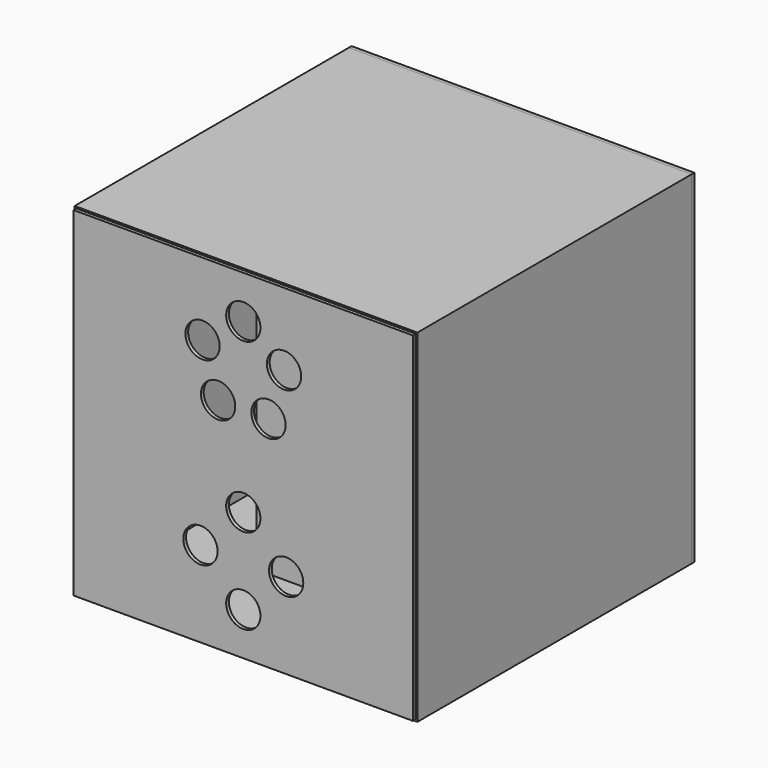
from build123d import *

# Parameters (mm, degrees)
F0_R      = 5.5
F1_DEPTH  = 19
F0_W      = 24.5
F0_H      = 25
F2_DEPTH  = 10
F3_DEPTH  = 60
F0_W_2    = 25
F0_H_2    = 0.5
F4_DEPTH  = 25
F5_D      = 10
F5_2_D    = 10
F5_3_D    = 10
F5_4_D    = 10
F5_5_D    = 10
F6_W      = 100
F6_H      = 100
F6_W_2    = 99
F6_H_2    = 99
F7_DEPTH  = 100
F8_W      = 99
F8_H      = 99
F8_R      = 5
F9_DEPTH  = 1
F10_W     = 100
F10_H     = 100
F11_DEPTH = 1
F13_R     = 5
F13_W     = 49.9103330076
F13_H     = 49.2593720555
F13_H_2   = 0.8928030729
F14_DEPTH = 5


# Not quite as in the source:
# - a pattern or mirror of a feature is missing from the dataset's text; its kind, count and spacing are read off the source's solid
# - a feature names something its author has since deleted; it is built from what else it names


with BuildPart() as f1:
    # F0 (on Front) → F1 (new body)
    with BuildSketch(Plane.XZ):
        with BuildLine():
            Line((-15.8034909498, 24.5), (-25, 24.5))
            Line((-25, 24.5), (-25, 0.5))
            Line((-25, 0.5), (0, 0.5))
            Line((0, 0.5), (0, 24.5))
            Line((0, 24.5), (-7.9729219576, 24.5))
            ThreePointArc((-7.9729219576, 24.5), (-11.8882064537, 22.8627124297), (-15.8034909498, 24.5))
        make_face()
        with Locations((-7.3473156537, 14.3872875703)):
            Circle(F0_R, mode=Mode.SUBTRACT)
        with BuildLine():
            Line((0, 49.5), (-25, 49.5))
            Line((-25, 49.5), (-25, 24.5))
            Line((-25, 24.5), (-15.8034909498, 24.5))
            ThreePointArc((-15.8034909498, 24.5), (-13.9757810358, 33.4511338317), (-6.3882064537, 28.3627124297))
            ThreePointArc((-6.3882064537, 28.3627124297), (-6.7997850517, 26.2751378476), (-7.9729219576, 24.5))
            Line((-7.9729219576, 24.5), (0, 24.5))
            Line((0, 24.5), (0, 31.5))
            ThreePointArc((0, 31.5), (-5.5, 37), (0, 42.5))
            Line((0, 42.5), (0, 49.5))
        make_face()
        with BuildLine():
            Line((25, 49.5), (0, 49.5))
            Line((0, 49.5), (0, 42.5))
            ThreePointArc((0, 42.5), (3.8890872965, 40.8890872965), (5.5, 37))
            ThreePointArc((5.5, 37), (3.8890872965, 33.1109127035), (0, 31.5))
            Line((0, 31.5), (0, 24.5))
            Line((0, 24.5), (7.9729219576, 24.5))
            ThreePointArc((7.9729219576, 24.5), (9.8006318716, 33.4511338317), (17.3882064537, 28.3627124297))
            ThreePointArc((17.3882064537, 28.3627124297), (16.9766278557, 26.2751378476), (15.8034909498, 24.5))
            Line((15.8034909498, 24.5), (25, 24.5))
            Line((25, 24.5), (25, 49.5))
        make_face()
        with BuildLine():
            Line((25, 0.5), (25, 24.5))
            Line((25, 24.5), (15.8034909498, 24.5))
            ThreePointArc((15.8034909498, 24.5), (11.8882064537, 22.8627124297), (7.9729219576, 24.5))
            Line((7.9729219576, 24.5), (0, 24.5))
            Line((0, 24.5), (0, 0.5))
            Line((0, 0.5), (25, 0.5))
        make_face()
        with Locations((7.3473156537, 14.3872875703)):
            Circle(F0_R, mode=Mode.SUBTRACT)
    extrude(amount=F1_DEPTH)

    # F0 (on Front) → F2 (join)
    with BuildSketch(Plane.XZ):
        with Locations((-37.25, 37)):
            Rectangle(F0_W, F0_H)
        Polygon((-25, 24.5), (-49.5, 24.5), (-49.5, 0), (-25, 0), (-25, 0.5), align=None)
        Polygon((-25, 0), (-49.5, 0), (-49.5, -24.5), (-25, -24.5), (-25, -0.5), align=None)
        with Locations((-37.25, -37)):
            Rectangle(F0_W, F0_H)
        with Locations((37.25, -37)):
            Rectangle(F0_W, F0_H)
        Polygon((49.5, 0), (25, 0), (25, -0.5), (25, -24.5), (49.5, -24.5), align=None)
        Polygon((49.5, 24.5), (25, 24.5), (25, 0.5), (25, 0), (49.5, 0), align=None)
        with Locations((37.25, 37)):
            Rectangle(F0_W, F0_H)
    extrude(amount=F2_DEPTH)

    # F0 (on Front) → F3 (join)
    with BuildSketch(Plane.XZ):
        with BuildLine():
            ThreePointArc((-6.3882064537, 28.3627124297), (-13.9757810358, 33.4511338317), (-15.8034909498, 24.5))
            Line((-15.8034909498, 24.5), (-7.9729219576, 24.5))
            ThreePointArc((-7.9729219576, 24.5), (-6.7997850517, 26.2751378476), (-6.3882064537, 28.3627124297))
        make_face()
        with BuildLine():
            Line((-7.9729219576, 24.5), (-15.8034909498, 24.5))
            ThreePointArc((-15.8034909498, 24.5), (-11.8882064537, 22.8627124297), (-7.9729219576, 24.5))
        make_face()
        with BuildLine():
            ThreePointArc((5.5, 37), (3.8890872965, 40.8890872965), (0, 42.5))
            Line((0, 42.5), (0, 31.5))
            ThreePointArc((0, 31.5), (3.8890872965, 33.1109127035), (5.5, 37))
        make_face()
        with BuildLine():
            Line((0, 31.5), (0, 42.5))
            ThreePointArc((0, 42.5), (-5.5, 37), (0, 31.5))
        make_face()
        with Locations((7.3473156537, 14.3872875703)):
            Circle(F0_R)
        with Locations((-7.3473156537, 14.3872875703)):
            Circle(F0_R)
    f3_solid = extrude(amount=F3_DEPTH)

    # F3_copies: F3 across plane
    add(f3_solid.mirror(Plane(origin=(0, 0, 0), x_dir=(0, 0, 1), z_dir=(1, 0, 0))))

    # F5 (through all)
    with Locations(Plane(origin=(0, 0, 0), x_dir=(1, 0, 0), z_dir=(0, 1, 0))):
        with Locations((-11.8882064537, -28.3627124297), (0, -37), (11.8882064537, -28.3627124297), (7.3473156537, -14.3872875703), (-7.3473156537, -14.3872875703), (0, 12), (-12.5, 24.5), (0, 37), (12.5, 24.5)):
            Hole(F5_D / 2)


with BuildPart() as f1b:
    # F0 (on Front) → F1, piece 2 (new body)
    with BuildSketch(Plane.XZ):
        with BuildLine():
            Line((-25, -0.5), (-25, -24.5))
            Line((-25, -24.5), (-18, -24.5))
            ThreePointArc((-18, -24.5), (-12.5, -19), (-7, -24.5))
            Line((-7, -24.5), (0, -24.5))
            Line((0, -24.5), (0, -17.5))
            ThreePointArc((0, -17.5), (-5.5, -12), (0, -6.5))
            Line((0, -6.5), (0, -0.5))
            Line((0, -0.5), (-25, -0.5))
        make_face()
        with BuildLine():
            Line((25, -0.5), (0, -0.5))
            Line((0, -0.5), (0, -6.5))
            ThreePointArc((0, -6.5), (3.8890872965, -8.1109127035), (5.5, -12))
            ThreePointArc((5.5, -12), (3.8890872965, -15.8890872965), (0, -17.5))
            Line((0, -17.5), (0, -24.5))
            Line((0, -24.5), (7, -24.5))
            ThreePointArc((7, -24.5), (12.5, -19), (18, -24.5))
            Line((18, -24.5), (25, -24.5))
            Line((25, -24.5), (25, -0.5))
        make_face()
        with BuildLine():
            Line((0, -42.5), (0, -49.5))
            Line((0, -49.5), (25, -49.5))
            Line((25, -49.5), (25, -24.5))
            Line((25, -24.5), (18, -24.5))
            ThreePointArc((18, -24.5), (12.5, -30), (7, -24.5))
            Line((7, -24.5), (0, -24.5))
            Line((0, -24.5), (0, -31.5))
            ThreePointArc((0, -31.5), (3.8890872965, -33.1109127035), (5.5, -37))
            ThreePointArc((5.5, -37), (3.8890872965, -40.8890872965), (0, -42.5))
        make_face()
        with BuildLine():
            Line((-18, -24.5), (-25, -24.5))
            Line((-25, -24.5), (-25, -49.5))
            Line((-25, -49.5), (0, -49.5))
            Line((0, -49.5), (0, -42.5))
            ThreePointArc((0, -42.5), (-5.5, -37), (0, -31.5))
            Line((0, -31.5), (0, -24.5))
            Line((0, -24.5), (-7, -24.5))
            ThreePointArc((-7, -24.5), (-12.5, -30), (-18, -24.5))
        make_face()
    extrude(amount=F1_DEPTH)


with BuildPart() as f3:
    # F0 (on Front) → F3, piece 2 (new body)
    with BuildSketch(Plane.XZ):
        with BuildLine():
            Line((0, -17.5), (0, -6.5))
            ThreePointArc((0, -6.5), (-5.5, -12), (0, -17.5))
        make_face()
        with BuildLine():
            ThreePointArc((5.5, -12), (3.8890872965, -8.1109127035), (0, -6.5))
            Line((0, -6.5), (0, -17.5))
            ThreePointArc((0, -17.5), (3.8890872965, -15.8890872965), (5.5, -12))
        make_face()
    extrude(amount=F3_DEPTH)

    # F5#2 (through all)
    with Locations(Plane(origin=(0, 0, 0), x_dir=(1, 0, 0), z_dir=(0, 1, 0))):
        with Locations((-11.8882064537, -28.3627124297), (0, -37), (11.8882064537, -28.3627124297), (7.3473156537, -14.3872875703), (-7.3473156537, -14.3872875703), (0, 12), (-12.5, 24.5), (0, 37), (12.5, 24.5)):
            Hole(F5_2_D / 2)


with BuildPart() as f3b:
    # F0 (on Front) → F3, piece 3 (new body)
    with BuildSketch(Plane.XZ):
        with BuildLine():
            Line((-7, -24.5), (-18, -24.5))
            ThreePointArc((-18, -24.5), (-12.5, -30), (-7, -24.5))
        make_face()
        with BuildLine():
            ThreePointArc((-7, -24.5), (-12.5, -19), (-18, -24.5))
            Line((-18, -24.5), (-7, -24.5))
        make_face()
    extrude(amount=F3_DEPTH)

    # F5#3 (through all)
    with Locations(Plane(origin=(0, 0, 0), x_dir=(1, 0, 0), z_dir=(0, 1, 0))):
        with Locations((-11.8882064537, -28.3627124297), (0, -37), (11.8882064537, -28.3627124297), (7.3473156537, -14.3872875703), (-7.3473156537, -14.3872875703), (0, 12), (-12.5, 24.5), (0, 37), (12.5, 24.5)):
            Hole(F5_3_D / 2)


with BuildPart() as f3c:
    # F0 (on Front) → F3, piece 4 (new body)
    with BuildSketch(Plane.XZ):
        with BuildLine():
            Line((18, -24.5), (7, -24.5))
            ThreePointArc((7, -24.5), (12.5, -30), (18, -24.5))
        make_face()
        with BuildLine():
            ThreePointArc((18, -24.5), (12.5, -19), (7, -24.5))
            Line((7, -24.5), (18, -24.5))
        make_face()
    extrude(amount=F3_DEPTH)

    # F5#4 (through all)
    with Locations(Plane(origin=(0, 0, 0), x_dir=(1, 0, 0), z_dir=(0, 1, 0))):
        with Locations((-11.8882064537, -28.3627124297), (0, -37), (11.8882064537, -28.3627124297), (7.3473156537, -14.3872875703), (-7.3473156537, -14.3872875703), (0, 12), (-12.5, 24.5), (0, 37), (12.5, 24.5)):
            Hole(F5_4_D / 2)


with BuildPart() as f3d:
    # F0 (on Front) → F3, piece 5 (new body)
    with BuildSketch(Plane.XZ):
        with BuildLine():
            ThreePointArc((0, -31.5), (-5.5, -37), (0, -42.5))
            Line((0, -42.5), (0, -31.5))
        make_face()
        with BuildLine():
            Line((0, -31.5), (0, -42.5))
            ThreePointArc((0, -42.5), (3.8890872965, -40.8890872965), (5.5, -37))
            ThreePointArc((5.5, -37), (3.8890872965, -33.1109127035), (0, -31.5))
        make_face()
    extrude(amount=F3_DEPTH)

    # F5#5 (through all)
    with Locations(Plane(origin=(0, 0, 0), x_dir=(1, 0, 0), z_dir=(0, 1, 0))):
        with Locations((-11.8882064537, -28.3627124297), (0, -37), (11.8882064537, -28.3627124297), (7.3473156537, -14.3872875703), (-7.3473156537, -14.3872875703), (0, 12), (-12.5, 24.5), (0, 37), (12.5, 24.5)):
            Hole(F5_5_D / 2)


with BuildPart() as f4:
    # F0 (on Front) → F4 (new body)
    with BuildSketch(Plane.XZ):
        with Locations((-12.5, -0.25)):
            Rectangle(F0_W_2, F0_H_2)
        with Locations((-12.5, 0.25)):
            Rectangle(F0_W_2, F0_H_2)
        with Locations((12.5, 0.25)):
            Rectangle(F0_W_2, F0_H_2)
        with Locations((12.5, -0.25)):
            Rectangle(F0_W_2, F0_H_2)
    extrude(amount=F4_DEPTH)


with BuildPart() as f7:
    # F6 (on Front) → F7 (new body)
    with BuildSketch(Plane.XZ):
        Rectangle(F6_W, F6_H)
        Rectangle(F6_W_2, F6_H_2, mode=Mode.SUBTRACT)
    extrude(amount=F7_DEPTH)


with BuildPart() as f9:
    # F8 (on face) → F9 (new body)
    with BuildSketch(Plane.XZ.offset(100)):
        Rectangle(F8_W, F8_H)
        with Locations((-12.5, -24.5)):
            Circle(F8_R, mode=Mode.SUBTRACT)
        with Locations((0, -37)):
            Circle(F8_R, mode=Mode.SUBTRACT)
        with Locations((12.5, -24.5)):
            Circle(F8_R, mode=Mode.SUBTRACT)
        with Locations((0, -12)):
            Circle(F8_R, mode=Mode.SUBTRACT)
        with Locations((-7.3473156537, 14.3872875703)):
            Circle(F8_R, mode=Mode.SUBTRACT)
        with Locations((-11.8882064537, 28.3627124297)):
            Circle(F8_R, mode=Mode.SUBTRACT)
        with Locations((7.3473156537, 14.3872875703)):
            Circle(F8_R, mode=Mode.SUBTRACT)
        with Locations((11.8882064537, 28.3627124297)):
            Circle(F8_R, mode=Mode.SUBTRACT)
        with Locations((0, 37)):
            Circle(F8_R, mode=Mode.SUBTRACT)
    extrude(amount=F9_DEPTH)


with BuildPart() as f11:
    # F10 (on Front) → F11 (new body)
    with BuildSketch(Plane.XZ):
        Rectangle(F10_W, F10_H)
    extrude(amount=-F11_DEPTH)


with BuildPart() as f14:
    # F13 (on offset) → F14 (new body)
    with BuildSketch(Plane.XZ.offset(60)):
        Polygon((24.9788202345, -0.2071894705), (24.9788202345, 49.4724996388), (-24.9788202345, 49.4724996388), (-24.9788202345, -0.2071894705), (-24.9551665038, -0.2071894705), (-24.9551665038, 0.6856136024), (24.9551665038, 0.6856136024), (24.9551665038, -0.2071894705), align=None)
        with Locations((-7.3473156537, 14.3872875703)):
            Circle(F13_R, mode=Mode.SUBTRACT)
        with Locations((-11.8882064537, 28.3627124297)):
            Circle(F13_R, mode=Mode.SUBTRACT)
        with Locations((7.3473156537, 14.3872875703)):
            Circle(F13_R, mode=Mode.SUBTRACT)
        with Locations((0, 37)):
            Circle(F13_R, mode=Mode.SUBTRACT)
        with Locations((11.8882064537, 28.3627124297)):
            Circle(F13_R, mode=Mode.SUBTRACT)
        with Locations((0, -24.8368754983)):
            Rectangle(F13_W, F13_H)
        with Locations((-12.5063573942, -24.4981031865)):
            Circle(F13_R, mode=Mode.SUBTRACT)
        with Locations((0, -36.9887426496)):
            Circle(F13_R, mode=Mode.SUBTRACT)
        with Locations((0, -12.0074609295)):
            Circle(F13_R, mode=Mode.SUBTRACT)
        with Locations((12.5, -24.5)):
            Circle(F13_R, mode=Mode.SUBTRACT)
        with Locations((0, 0.2392120659)):
            Rectangle(F13_W, F13_H_2)
    extrude(amount=F14_DEPTH)


solid = Compound([f1.part, f1b.part, f3.part, f3b.part, f3c.part, f3d.part, f4.part, f7.part, f9.part, f11.part, f14.part])
